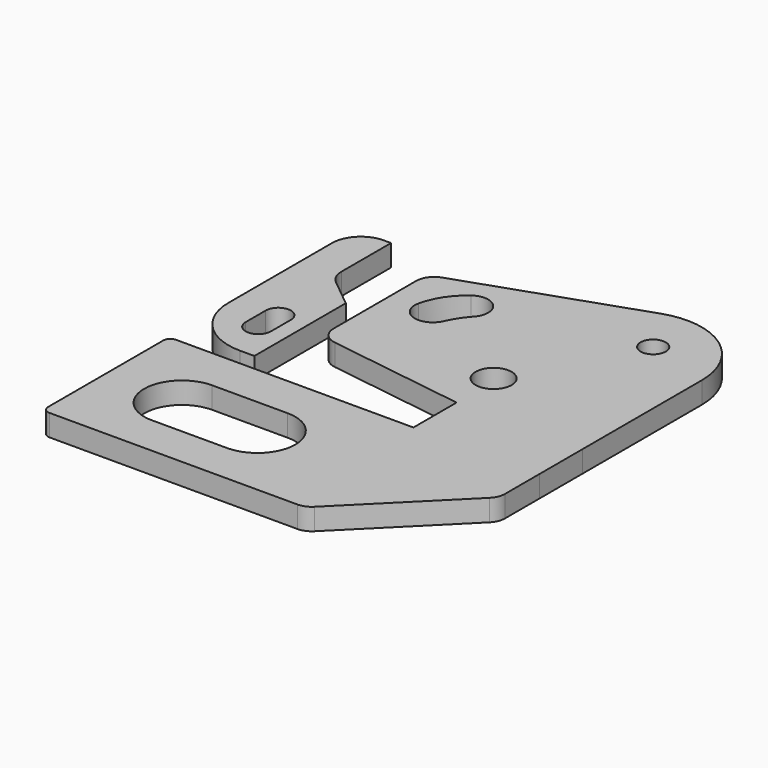
from build123d import *

# Parameters (mm, degrees)
F0_R     = 5
F0_R_2   = 3.500004939
F1_DEPTH = 6


# Not quite as in the source:
# - a feature names something its author has since deleted; it is built from what else it names


with BuildPart() as f1:
    # F0 (on Top) → F1 (new body)
    with BuildSketch(Plane.XY):
        with BuildLine():
            Line((16.1606259644, -4.6810654402), (-49.79929021, -4.6810654402))
            ThreePointArc((-49.79929021, -4.6810654402), (-51.2135037724, -5.2668518778), (-51.79929021, -6.6810654402))
            Line((-51.79929021, -6.6810654402), (-51.79929021, -46.6810654402))
            ThreePointArc((-51.79929021, -46.6810654402), (-51.2135037724, -48.0952790026), (-49.79929021, -48.6810654402))
            Line((-49.79929021, -48.6810654402), (19.1248844436, -48.6810654402))
            ThreePointArc((19.1248844436, -48.6810654402), (21.036564704, -48.3011821684), (22.6577588236, -47.219256873))
            Line((22.6577588236, -47.219256873), (49.73358417, -20.1841199958))
            ThreePointArc((49.73358417, -20.1841199958), (50.8193877339, -18.5610823557), (51.20070979, -16.6459285629))
            Line((51.20070979, -16.6459285629), (51.20070979, -4.6810654402))
            Line((51.20070979, -4.6810654402), (51.1966860054, 10.3189345598))
            Line((51.1966860054, 10.3189345598), (51.1855687764, 51.762116243))
            ThreePointArc((51.1855687764, 51.762116243), (42.7975370702, 68.0405532426), (24.6744211265, 70.6671966416))
            Line((24.6744211265, 70.6671966416), (-23.1247563194, 54.2092270392))
            ThreePointArc((-23.1247563194, 54.2092270392), (-25.5108689481, 52.3786930394), (-26.4153077682, 49.5105266177))
            Line((-26.4153077682, 49.5105266177), (-26.4153077682, 20.7971311183))
            ThreePointArc((-26.4153077682, 20.7971311183), (-25.1454430856, 17.4675529898), (-21.9808715626, 15.8292203306))
            Line((-21.9808715626, 15.8292203306), (16.1606259644, 10.3189345598))
            Line((16.1606259644, 10.3189345598), (16.1606259644, -4.6810654402))
        make_face()
        with BuildLine():
            ThreePointArc((-30.3327057958, -37.5000230521), (-40.8327057958, -27.0000230521), (-30.3327057958, -16.5000230521))
            Line((-30.3327057958, -16.5000230521), (-9.3327057958, -16.5000230521))
            ThreePointArc((-9.3327057958, -16.5000230521), (1.1672942042, -27.0000230521), (-9.3327057958, -37.5000230521))
            Line((-9.3327057958, -37.5000230521), (-30.3327057958, -37.5000230521))
        make_face(mode=Mode.SUBTRACT)
        with BuildLine():
            ThreePointArc((-9.9462399779, 38.4116526327), (-16.0676429129, 35.6625089912), (-19.4117133222, 41.4802884432))
            ThreePointArc((-19.4117133222, 41.4802884432), (-17.0396688443, 47.1598668703), (-12.8037057075, 51.6253816691))
            ThreePointArc((-12.8037057075, 51.6253816691), (-6.1306487798, 50.9185041026), (-6.1706380254, 44.2082309699))
            ThreePointArc((-6.1706380254, 44.2082309699), (-8.2969904977, 41.4653223451), (-9.9462399779, 38.4116526327))
        make_face(mode=Mode.SUBTRACT)
        with Locations((15.3547544032, 24.1966232508)):
            Circle(F0_R, mode=Mode.SUBTRACT)
        with Locations((33.151564105, 57.4042351962)):
            Circle(F0_R_2, mode=Mode.SUBTRACT)
    extrude(amount=F1_DEPTH)


with BuildPart() as f1b:
    # F0 (on Top) → F1, piece 2 (new body)
    with BuildSketch(Plane.XY):
        with BuildLine():
            Line((-31.79929021, 0), (-31.79929021, 31.7654939741))
            Line((-31.79929021, 31.7654939741), (-39.5897412392, 38.1144208726))
            ThreePointArc((-39.5897412392, 38.1144208726), (-41.2188246077, 40.1908780974), (-41.79929021, 42.7654939741))
            Line((-41.79929021, 42.7654939741), (-41.79929021, 60))
            Line((-41.79929021, 60), (-43.79929021, 60))
            ThreePointArc((-43.79929021, 60), (-49.4561444595, 57.6568542495), (-51.79929021, 52))
            Line((-51.79929021, 52), (-51.79929021, 16))
            ThreePointArc((-51.79929021, 16), (-47.112998709, 4.686291501), (-35.79929021, 0))
            Line((-35.79929021, 0), (-31.79929021, 0))
        make_face()
        with BuildLine():
            ThreePointArc((-43.2216169983, 18.230368793), (-39.7216169983, 21.730368793), (-36.2216169983, 18.230368793))
            Line((-36.2216169983, 18.230368793), (-36.2216169983, 11.2746311097))
            ThreePointArc((-36.2216169983, 11.2746311097), (-39.7216169983, 7.7746311097), (-43.2216169983, 11.2746311097))
            Line((-43.2216169983, 11.2746311097), (-43.2216169983, 18.230368793))
        make_face(mode=Mode.SUBTRACT)
    extrude(amount=F1_DEPTH)


with BuildPart() as f2_1:
    # F2: copy of F1b
    add(f1b.part)


solid = Compound([f1.part, f1b.part, f2_1.part])
